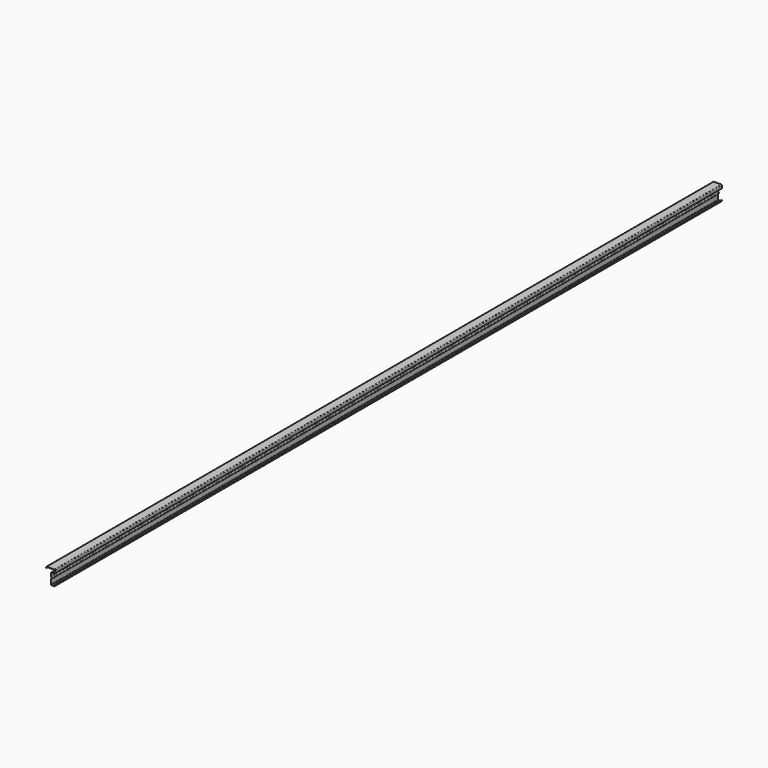
from build123d import *

# Parameters (mm, degrees)
F1_DEPTH = 5000


# Not quite as in the source:
# - ends of sketch curves that miss each other by under 0.0002 mm in the source are joined


with BuildPart() as f1:
    # F0 (on Front) → F1 (new body)
    with BuildSketch(Plane.XZ):
        with BuildLine():
            Line((26.2818114252, -40.2073050281), (26.2818114252, -36.177426882))
            Line((26.2818114252, -36.177426882), (24.7925087778, -36.177426882))
            Line((24.7925087778, -36.177426882), (24.7925087778, -40.2073046339))
            ThreePointArc((24.7925087778, -40.2073046339), (23.9714139143, -42.1896029892), (21.9891155591, -43.0106978526))
            Line((21.9891155591, -43.0106978526), (6.9208770086, -43.0106978526))
            ThreePointArc((6.9208770086, -43.0106978526), (4.9385786534, -42.1896029892), (4.1174837899, -40.2073046339))
            Line((4.1174837899, -40.2073046339), (4.1174837899, -30.6058300818))
            Line((4.1174837899, -30.6058300818), (4.1174837899, -14.0251837989))
            ThreePointArc((4.1174837899, -14.0251837989), (4.4509143771, -12.3489149315), (5.4004443607, -10.9278427721))
            Line((5.4004443607, -10.9278427721), (7.6621440673, -8.6661430321))
            ThreePointArc((7.6621440673, -8.6661430321), (8.9194384176, -5.6307558244), (7.662136908, -2.5953614834))
            Line((7.662136908, -2.5953614834), (5.4004444754, -0.3336690558))
            ThreePointArc((5.4004444754, -0.3336690558), (4.4509144127, 1.0874031659), (4.1174837899, 2.7636721191))
            Line((4.1174837899, 2.7636721191), (4.1174837899, 19.444672608))
            ThreePointArc((4.1174837899, 19.444672608), (4.9385786534, 21.4269709633), (6.9208770086, 22.2480658267))
            Line((6.9208770086, 22.2480658267), (21.9891155591, 22.2480658267))
            ThreePointArc((21.9891155591, 22.2480658267), (25.0245099156, 23.5053673363), (26.2818114252, 26.5407616928))
            Line((26.2818114252, 26.5407616928), (26.2818114252, 40.2073036339))
            ThreePointArc((26.2818114252, 40.2073036339), (25.0245099156, 43.2426979904), (21.9891155591, 44.4999995))
            Line((21.9891155591, 44.4999995), (-21.9891155591, 44.4999995))
            ThreePointArc((-21.9891155591, 44.4999995), (-25.0245099156, 43.2426979904), (-26.2818114252, 40.2073036339))
            Line((-26.2818114252, 40.2073036339), (-26.2818114252, 36.177425882))
            Line((-26.2818114252, 36.177425882), (-24.7925087778, 36.177425882))
            Line((-24.7925087778, 36.177425882), (-24.7925087778, 40.2073036339))
            ThreePointArc((-24.7925087778, 40.2073036339), (-23.9714139143, 42.1896019892), (-21.9891155591, 43.0106968526))
            Line((-21.9891155591, 43.0106968526), (21.9891155591, 43.0106968526))
            ThreePointArc((21.9891155591, 43.0106968526), (23.9714139143, 42.1896019892), (24.7925087778, 40.2073036339))
            Line((24.7925087778, 40.2073036339), (24.7925087778, 26.5407616928))
            ThreePointArc((24.7925087778, 26.5407616928), (23.9714139143, 24.5584633375), (21.9891155591, 23.7373684741))
            Line((21.9891155591, 23.7373684741), (6.9208770086, 23.7373684741))
            ThreePointArc((6.9208770086, 23.7373684741), (3.8854826521, 22.4800669645), (2.6281811425, 19.444672608))
            Line((2.6281811425, 19.444672608), (2.6281811425, 2.8725354557))
            ThreePointArc((2.6281811425, 2.8725354557), (3.0949839305, 0.525758642), (4.4243261563, -1.4637426783))
            Line((4.4243261563, -1.4637426783), (6.6090409069, -3.6484574844))
            ThreePointArc((6.6090409069, -3.6484574844), (7.4301357701, -5.6307558399), (6.6090409067, -7.6130541952))
            Line((6.6090409067, -7.6130541952), (4.4243263037, -9.7977687547))
            ThreePointArc((4.4243263037, -9.7977687547), (3.0949840701, -11.7872699409), (2.6281811425, -14.1340466099))
            Line((2.6281811425, -14.1340466099), (2.6281811425, -30.4969672709))
            Line((2.6281811425, -30.4969672709), (2.6281811425, -40.2073046339))
            ThreePointArc((2.6281811425, -40.2073046339), (3.8854826521, -43.2426989904), (6.9208770086, -44.5000005))
            Line((6.9208770086, -44.5000005), (21.9891155591, -44.5000005))
            ThreePointArc((21.9891155591, -44.5000005), (25.0245099156, -43.2426989904), (26.2818114252, -40.2073050281))
        make_face()
    extrude(amount=-F1_DEPTH)


solid = f1.part
